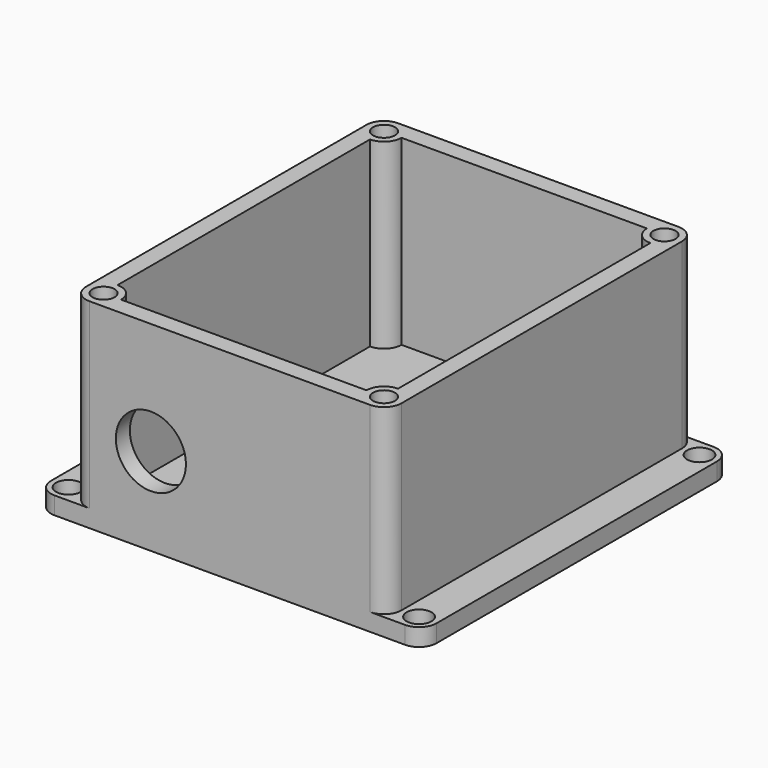
from build123d import *

# Parameters (mm, degrees)
F0_W          = 69.85
F0_H          = 69.85
F1_DEPTH      = 3.175
F2_R          = 3.175
F3_R          = 2.2499955
F4_DEPTH      = 25.4
F4_DEPTH_BACK = 101
F6_DEPTH      = 25.4
F7_R          = 1.999996
F8_DEPTH      = 6.35
F9_R          = 6.35
F10_DEPTH     = 3.175
F11_DEPTH     = 7.62


# Not quite as in the source:
# - an extrude ends at something that could not be found from the text; its depth is read off the source's solid


with BuildPart() as f1:
    # F0 (on Top) → F1 (new body)
    with BuildSketch(Plane.XY):
        Rectangle(F0_W, F0_H)
    extrude(amount=F1_DEPTH)

    # F2
    f2_edges = [f1.edges().sort_by_distance(p)[0] for p in [
        (-34.925, -34.925, 1.5875),
        (34.925, -34.925, 1.5875),
        (34.925, 34.925, 1.5875),
        (-34.925, 34.925, 1.5875),
    ]]
    fillet(f2_edges, radius=F2_R)

    # F3 (on face) → F4 (cut, two sides)
    with BuildSketch(Plane.XY.offset(3.175)) as f4_sk:
        with Locations((-31.75, 31.75)):
            Circle(F3_R)
        with Locations((31.75, 31.75)):
            Circle(F3_R)
        with Locations((31.75, -31.75)):
            Circle(F3_R)
        with Locations((-31.75, -31.75)):
            Circle(F3_R)
    extrude(amount=-F4_DEPTH, mode=Mode.SUBTRACT)
    extrude(f4_sk.sketch, amount=F4_DEPTH_BACK, mode=Mode.SUBTRACT)

    # F5 (on face) → F6 (join)
    with BuildSketch(Plane.XY.offset(3.175)):
        with BuildLine():
            Line((25.4, 34.925), (-25.4, 34.925))
            ThreePointArc((-25.4, 34.925), (-27.6450640303, 33.9950640303), (-28.575, 31.75))
            Line((-28.575, 31.75), (-28.575, -31.75))
            ThreePointArc((-28.575, -31.75), (-27.6450640303, -33.9950640303), (-25.4, -34.925))
            Line((-25.4, -34.925), (25.4, -34.925))
            ThreePointArc((25.4, -34.925), (27.6450640303, -33.9950640303), (28.575, -31.75))
            Line((28.575, -31.75), (28.575, 31.75))
            ThreePointArc((28.575, 31.75), (27.6450640303, 33.9950640303), (25.4, 34.925))
        make_face()
        with BuildLine():
            ThreePointArc((-25.4, 28.575), (-23.1549359697, 29.5049359697), (-22.225, 31.75))
            Line((-22.225, 31.75), (22.225, 31.75))
            ThreePointArc((22.225, 31.75), (23.1549359697, 29.5049359697), (25.4, 28.575))
            Line((25.4, 28.575), (25.4, -28.575))
            ThreePointArc((25.4, -28.575), (23.1549359697, -29.5049359697), (22.225, -31.75))
            Line((22.225, -31.75), (-22.225, -31.75))
            ThreePointArc((-22.225, -31.75), (-23.1549359697, -29.5049359697), (-25.4, -28.575))
            Line((-25.4, -28.575), (-25.4, 28.575))
        make_face(mode=Mode.SUBTRACT)
    extrude(amount=F6_DEPTH)

    # F7 (on face) → F8 (cut)
    with BuildSketch(Plane.XY.offset(28.575)):
        with Locations((-25.4, 31.75)):
            Circle(F7_R)
        with Locations((25.4, 31.75)):
            Circle(F7_R)
        with Locations((25.4, -31.75)):
            Circle(F7_R)
        with Locations((-25.4, -31.75)):
            Circle(F7_R)
    extrude(amount=-F8_DEPTH, mode=Mode.SUBTRACT)

    # F9 (on face) → F10 (cut, through all)
    with BuildSketch(Plane.XZ.offset(34.925)):
        with Locations((-14.2875, 15.875)):
            Circle(F9_R)
    extrude(amount=-F10_DEPTH, mode=Mode.SUBTRACT)

    # F11 (add): a face of the model
    f11_faces = [f1.faces().sort_by_distance(p)[0] for p in [
        (0, 34.0224954294, 28.575),
    ]]
    extrude(f11_faces, amount=F11_DEPTH)


solid = f1.part
